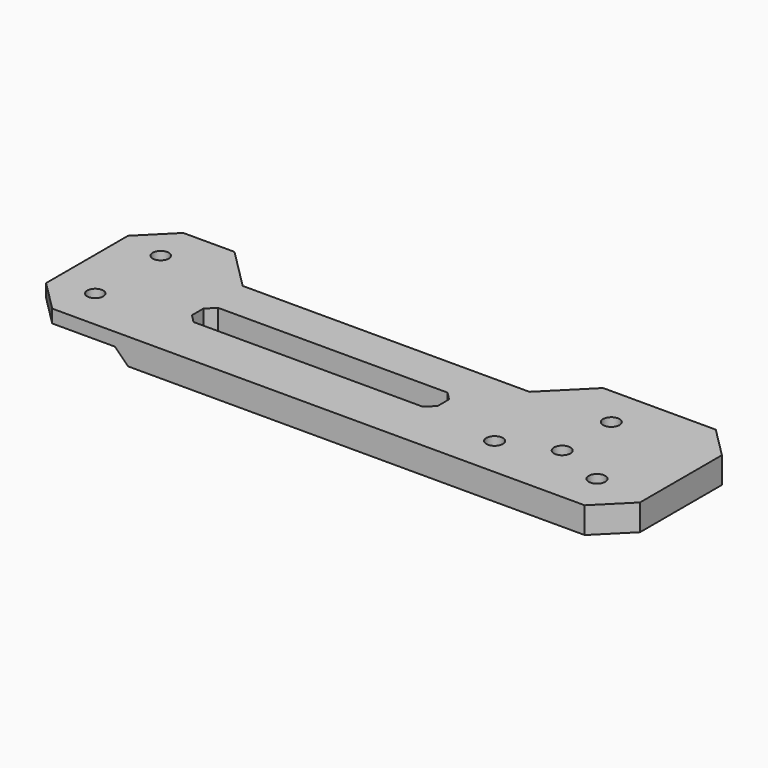
from build123d import *

# Parameters (mm, degrees)
F0_W      = 184.15
F0_H      = 50.8
F1_DEPTH  = 8.128
F3_D      = 5.1054
F6_D      = 4.9784
F7_W      = 76.2
F7_H      = 9.525
F8_DEPTH  = 8.129
F9_SIZE   = 9.525
F10_SIZE  = 2.54
F15_DEPTH = 25.4
F17_D     = 5.1054
F18_R     = 2.4892
F19_DEPTH = 4.064
F20_SIZE  = 4.06399


# Not quite as in the source:
# - a fillet or chamfer is up to 0.001 mm smaller than in the source, because OpenCascade refuses the exact size
# - a feature names something its author has since deleted; it is built from what else it names


with BuildPart() as f1:
    # F0 (on Top) → F1 (new body)
    with BuildSketch(Plane.XY):
        Rectangle(F0_W, F0_H)
    extrude(amount=F1_DEPTH)

    # F3 (through all)
    with Locations(Plane.XY.offset(8.128)):
        with Locations((-60.325, 12.7), (-76.2, -12.7), (-44.45, -12.7)):
            Hole(F3_D / 2)

    # F6 (through all)
    with Locations(Plane.XY.offset(8.128)):
        with Locations((79.375, 12.7), (79.375, -12.7)):
            Hole(F6_D / 2)

    # F7 (on face) → F8 (cut, through all)
    with BuildSketch(Plane.XY.offset(8.128)):
        Polygon((66.675, 25.4), (-47.625, 25.4), (-34.925, 12.7), (53.975, 12.7), align=None)
        with Locations((15.875, -4.7625)):
            Rectangle(F7_W, F7_H)
    extrude(amount=-F8_DEPTH, mode=Mode.SUBTRACT)

    # F9
    f9_edges = [f1.edges().sort_by_distance(p)[0] for p in [
        (-92.075, -25.4, 4.064),
        (-92.075, 25.4, 4.064),
        (92.075, -25.4, 4.064),
        (92.075, 25.4, 4.064),
    ]]
    chamfer(f9_edges, length=F9_SIZE)

    # F10
    f10_edges = [f1.edges().sort_by_distance(p)[0] for p in [
        (-22.225, 0, 4.064),
        (-22.225, -9.525, 4.064),
        (53.975, 0, 4.064),
        (53.975, -9.525, 4.064),
    ]]
    chamfer(f10_edges, length=F10_SIZE)


with BuildPart() as f13_1:
    # F13: instance of F1
    add(f1.part.mirror(Plane(origin=(92.075, 0, 4.064), x_dir=(0, 1, 0), z_dir=(1, 0, 0))))

    # F17 (through all)
    with Locations(Plane.XY.offset(8.128)):
        with Locations((244.475, -6.35)):
            Hole(F17_D / 2)

    # F18 (on face) → F19 (cut)
    with BuildSketch(Plane(origin=(0, 0, 0), x_dir=(1, 0, 0), z_dir=(0, 0, -1))):
        Polygon((125.095, 25.4), (117.475, 25.4), (101.6, 25.4), (92.075, 15.875), (92.075, -15.875), (101.6, -25.4), (117.475, -25.4), (125.095, -17.78), align=None)
        with Locations((104.775, -12.7)):
            Circle(F18_R, mode=Mode.SUBTRACT)
        with Locations((104.775, 12.7)):
            Circle(F18_R, mode=Mode.SUBTRACT)
    extrude(amount=-F19_DEPTH, mode=Mode.SUBTRACT)

    # F20 (size 4.064 in the source; OpenCascade refuses exactly that, so slightly less here)
    f20_edges = [f13_1.edges().sort_by_distance(p)[0] for p in [
        (125.095, -3.81, 4.064),
    ]]
    chamfer(f20_edges, length=F20_SIZE)


with BuildPart() as f1_1:
    add(f1.part)

    # F14 (on face) → F15 (cut)
    with BuildSketch(Plane.XY.offset(8.128)):
        Polygon((-100.5587801337, -25.4), (92.075, -25.4), (92.075, -15.875), (92.075, 15.875), (92.075, 34.0131297708), (-100.5587801337, 34.0131297708), align=None)
    extrude(amount=-F15_DEPTH, mode=Mode.SUBTRACT)


solid = f13_1.part
